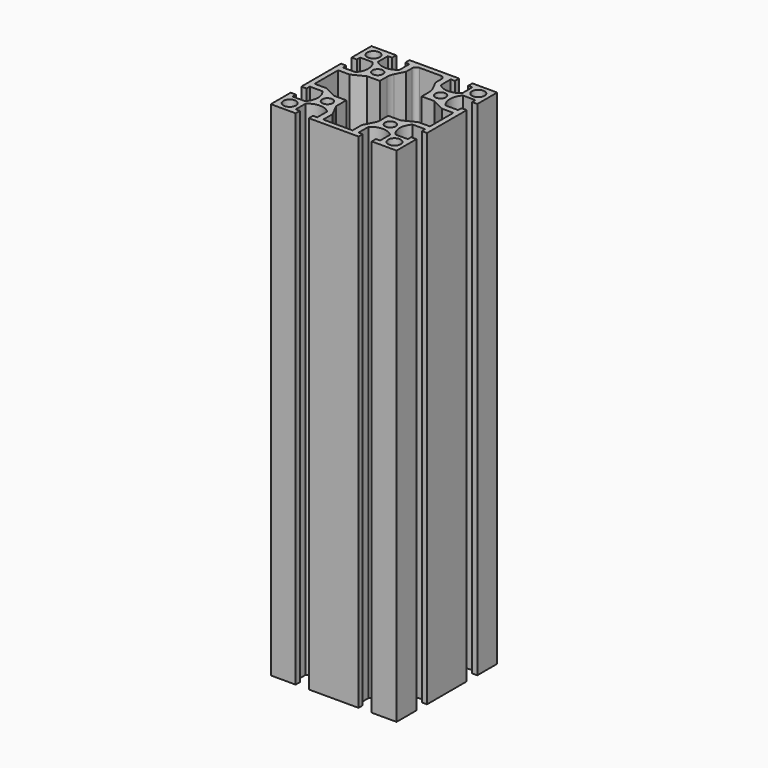
from build123d import *

# Parameters (mm, degrees)
F0_R     = 3
F0_R_2   = 2.5
F1_DEPTH = 240
F2_R     = 2
F3_R     = 7


# Not quite as in the source:
# - a feature names something its author has since deleted; it is built from what else it names


with BuildPart() as f1:
    # F0 (on Top) → F1 (new body)
    with BuildSketch(Plane.XY):
        with BuildLine():
            Line((18.15, -30), (30, -30))
            Line((30, -30), (30, -18.15))
            Line((30, -18.15), (27.5, -18.15))
            Line((27.5, -18.15), (27.5, -20.15))
            Line((27.5, -20.15), (21.5477069044, -20.15))
            ThreePointArc((21.5477069044, -20.15), (19.5, -15), (21.5477069044, -9.85))
            Line((21.5477069044, -9.85), (27.5, -9.85))
            Line((27.5, -9.85), (27.5, -11.85))
            Line((27.5, -11.85), (30, -11.85))
            Line((30, -11.85), (30, 11.85))
            Line((30, 11.85), (27.5, 11.85))
            Line((27.5, 11.85), (27.5, 9.85))
            Line((27.5, 9.85), (21.5477069044, 9.85))
            ThreePointArc((21.5477069044, 9.85), (19.5, 15), (21.5477069044, 20.15))
            Line((21.5477069044, 20.15), (27.5, 20.15))
            Line((27.5, 20.15), (27.5, 18.15))
            Line((27.5, 18.15), (30, 18.15))
            Line((30, 18.15), (30, 30))
            Line((30, 30), (18.15, 30))
            Line((18.15, 30), (18.15, 27.5))
            Line((18.15, 27.5), (20.15, 27.5))
            Line((20.15, 27.5), (20.15, 21.5477069044))
            ThreePointArc((20.15, 21.5477069044), (15, 19.5), (9.85, 21.5477069044))
            Line((9.85, 21.5477069044), (9.85, 27.5))
            Line((9.85, 27.5), (11.85, 27.5))
            Line((11.85, 27.5), (11.85, 30))
            Line((11.85, 30), (-11.85, 30))
            Line((-11.85, 30), (-11.85, 27.5))
            Line((-11.85, 27.5), (-9.85, 27.5))
            Line((-9.85, 27.5), (-9.85, 21.5477069044))
            ThreePointArc((-9.85, 21.5477069044), (-15, 19.5), (-20.15, 21.5477069044))
            Line((-20.15, 21.5477069044), (-20.15, 27.5))
            Line((-20.15, 27.5), (-18.15, 27.5))
            Line((-18.15, 27.5), (-18.15, 30))
            Line((-18.15, 30), (-30, 30))
            Line((-30, 30), (-30, 18.15))
            Line((-30, 18.15), (-27.5, 18.15))
            Line((-27.5, 18.15), (-27.5, 20.15))
            Line((-27.5, 20.15), (-21.5477069044, 20.15))
            ThreePointArc((-21.5477069044, 20.15), (-19.5, 15), (-21.5477069044, 9.85))
            Line((-21.5477069044, 9.85), (-27.5, 9.85))
            Line((-27.5, 9.85), (-27.5, 11.85))
            Line((-27.5, 11.85), (-30, 11.85))
            Line((-30, 11.85), (-30, -11.85))
            Line((-30, -11.85), (-27.5, -11.85))
            Line((-27.5, -11.85), (-27.5, -9.85))
            Line((-27.5, -9.85), (-21.5477069044, -9.85))
            ThreePointArc((-21.5477069044, -9.85), (-19.5, -15), (-21.5477069044, -20.15))
            Line((-21.5477069044, -20.15), (-27.5, -20.15))
            Line((-27.5, -20.15), (-27.5, -18.15))
            Line((-27.5, -18.15), (-30, -18.15))
            Line((-30, -18.15), (-30, -30))
            Line((-30, -30), (-18.15, -30))
            Line((-18.15, -30), (-18.15, -27.5))
            Line((-18.15, -27.5), (-20.15, -27.5))
            Line((-20.15, -27.5), (-20.15, -21.5477069044))
            ThreePointArc((-20.15, -21.5477069044), (-15, -19.5), (-9.85, -21.5477069044))
            Line((-9.85, -21.5477069044), (-9.85, -27.5))
            Line((-9.85, -27.5), (-11.85, -27.5))
            Line((-11.85, -27.5), (-11.85, -30))
            Line((-11.85, -30), (11.85, -30))
            Line((11.85, -30), (11.85, -27.5))
            Line((11.85, -27.5), (9.85, -27.5))
            Line((9.85, -27.5), (9.85, -21.5477069044))
            ThreePointArc((9.85, -21.5477069044), (15, -19.5), (20.15, -21.5477069044))
            Line((20.15, -21.5477069044), (20.15, -27.5))
            Line((20.15, -27.5), (18.15, -27.5))
            Line((18.15, -27.5), (18.15, -30))
        make_face()
        with Locations((-25, -25)):
            Circle(F0_R, mode=Mode.SUBTRACT)
        with Locations((-15, -15)):
            Circle(F0_R_2, mode=Mode.SUBTRACT)
        with Locations((25, -25)):
            Circle(F0_R, mode=Mode.SUBTRACT)
        with Locations((15, -15)):
            Circle(F0_R_2, mode=Mode.SUBTRACT)
        with Locations((-25, 25)):
            Circle(F0_R, mode=Mode.SUBTRACT)
        with Locations((-15, 15)):
            Circle(F0_R_2, mode=Mode.SUBTRACT)
        Polygon((-7, 22), (-7, 27.5), (0, 27.5), (7, 27.5), (7, 22), (10, 16), (10, 10), (16, 10), (22, 7), (27.5, 7), (27.5, 0), (27.5, -7), (22, -7), (16, -10), (10, -10), (10, -16), (7, -22), (7, -27.5), (0, -27.5), (-7, -27.5), (-7, -22), (-10, -16), (-10, -10), (-16, -10), (-22, -7), (-27.5, -7), (-27.5, 0), (-27.5, 7), (-22, 7), (-16, 10), (-10, 10), (-10, 16), align=None, mode=Mode.SUBTRACT)
        with Locations((15, 15)):
            Circle(F0_R_2, mode=Mode.SUBTRACT)
        with Locations((25, 25)):
            Circle(F0_R, mode=Mode.SUBTRACT)
    extrude(amount=F1_DEPTH)

    # F2
    f2_edges = [f1.edges().sort_by_distance(p)[0] for p in [
        (-7, 27.5, 120),
        (7, 27.5, 120),
    ]]
    fillet(f2_edges, radius=F2_R)

    # F3
    f3_edges = [f1.edges().sort_by_distance(p)[0] for p in [
        (-10, 16, 120),
        (10, 16, 120),
    ]]
    fillet(f3_edges, radius=F3_R)


solid = f1.part
